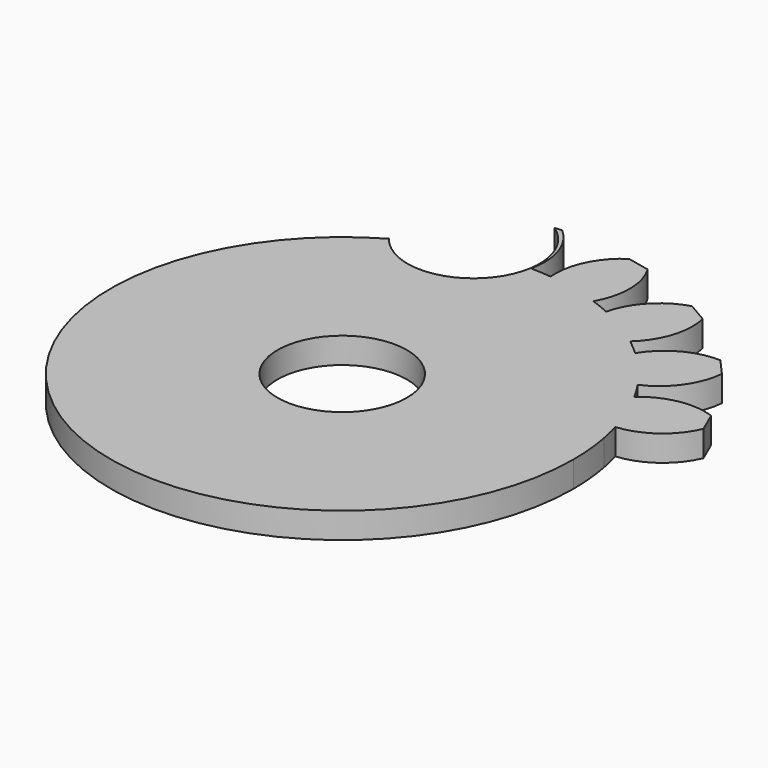
from build123d import *

# Parameters (mm, degrees)
F2_R     = 2.5
F3_DEPTH = 1


# Not quite as in the source:
# - a feature of the source that left no trace in its solid (it failed there, or was rolled back) is left out


with BuildPart() as f3:
    # F2 (on Top) → F3 (new body)
    with BuildSketch(Plane.XY):
        with BuildLine():
            ThreePointArc((-0.9522931143, 11.4531284813), (-0.0520635974, 10.3538099613), (0.1218940174, 8.943613826))
            ThreePointArc((0.1218940174, 8.943613826), (0.1337416353, 8.9434445039), (0.1455890186, 8.9432594873))
            ThreePointArc((0.1455890186, 8.9432594873), (0.0799521539, 10.3250380062), (-0.6817601701, 11.4797736507))
            Line((-0.6817601701, 11.4797736507), (-0.9522931143, 11.4531284813))
        make_face()
        with BuildLine():
            ThreePointArc((-4.4173624076, 7.7775314708), (-4.4995685223, -7.7302632253), (8.9444444444, 0))
            ThreePointArc((8.9444444444, 0), (8.9053271725, 0.8356041947), (8.7883175045, 1.6638995942))
            ThreePointArc((8.7883175045, 1.6638995942), (8.7057555111, 2.0525368209), (8.6060160514, 2.4371241541))
            ThreePointArc((8.6060160514, 2.4371241541), (8.2679218833, 3.4124117792), (7.8197142384, 4.3422523705))
            ThreePointArc((7.8197142384, 4.3422523705), (7.6211518715, 4.6820007018), (7.4078378155, 5.0126864374))
            ThreePointArc((7.4078378155, 5.0126864374), (6.7776596323, 5.8366442695), (6.0563228133, 6.5820999993))
            ThreePointArc((6.0563228133, 6.5820999993), (5.761965129, 6.84126043), (5.4565297326, 7.0872681406))
            ThreePointArc((5.4565297326, 7.0872681406), (4.5991510413, 7.6714337721), (3.6798961663, 8.1523892587))
            ThreePointArc((3.6798961663, 8.1523892587), (3.3179634912, 8.306275019), (2.9496159434, 8.4441016222))
            ThreePointArc((2.9496159434, 8.4441016222), (1.9566672267, 8.7278026893), (0.937636324, 8.8951629858))
            ThreePointArc((0.937636324, 8.8951629858), (0.542146294, 8.9279988696), (0.1455890186, 8.9432594873))
            ThreePointArc((0.1455890186, 8.9432594873), (0.1337416353, 8.9434445039), (0.1218940174, 8.943613826))
            ThreePointArc((0.1218940174, 8.943613826), (-1.7655892516, 6.8729814141), (-4.4173624076, 7.7775314708))
        make_face()
        Circle(F2_R, mode=Mode.SUBTRACT)
        with BuildLine():
            ThreePointArc((7.8197142384, 4.3422523705), (8.2679218833, 3.4124117792), (8.6060160514, 2.4371241541))
            ThreePointArc((8.6060160514, 2.4371241541), (9.8961633699, 2.9277974972), (10.7564598893, 4.0072095278))
            Line((10.7564598893, 4.0072095278), (10.398401005, 4.8258001529))
            ThreePointArc((10.398401005, 4.8258001529), (9.0439881545, 4.931031832), (7.8197142384, 4.3422523705))
        make_face()
        with BuildLine():
            ThreePointArc((6.0563228133, 6.5820999993), (6.7776596323, 5.8366442695), (7.4078378155, 5.0126864374))
            ThreePointArc((7.4078378155, 5.0126864374), (8.4689810733, 5.8780879937), (8.9469442237, 7.1612466333))
            Line((8.9469442237, 7.1612466333), (8.3534515739, 7.8291263012))
            ThreePointArc((8.3534515739, 7.8291263012), (7.0378063332, 7.5133903393), (6.0563228133, 6.5820999993))
        make_face()
        with BuildLine():
            ThreePointArc((3.6798961663, 8.1523892587), (4.5991510413, 7.6714337721), (5.4565297326, 7.0872681406))
            ThreePointArc((5.4565297326, 7.0872681406), (6.194311581, 8.236914632), (6.251341492, 9.6017430828))
            Line((6.251341492, 9.6017430828), (5.4805102725, 10.0535350783))
            ThreePointArc((5.4805102725, 10.0535350783), (4.3249499065, 9.344717804), (3.6798961663, 8.1523892587))
        make_face()
        with BuildLine():
            ThreePointArc((2.0608006124, 11.2812858546), (1.1761963647, 10.2402731247), (0.937636324, 8.8951629858))
            ThreePointArc((0.937636324, 8.8951629858), (1.9566672267, 8.7278026893), (2.9496159434, 8.4441016222))
            ThreePointArc((2.9496159434, 8.4441016222), (3.3010678965, 9.7691415234), (2.9335160712, 11.08980608))
            Line((2.9335160712, 11.08980608), (2.0608006124, 11.2812858546))
        make_face()
    extrude(amount=F3_DEPTH)


solid = f3.part
